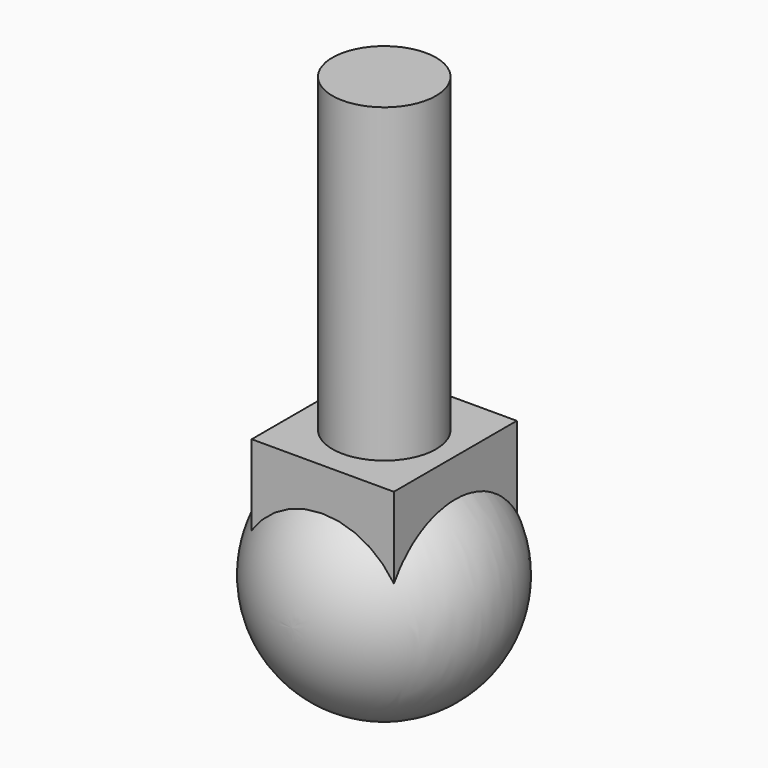
from build123d import *

# Parameters (mm, degrees)
F2_W      = 80.9100866318
F2_H      = 87.9881680012
F5_R      = 35.3495227498
F6_DEPTH  = 299.399793148
F9_W      = 97.0188975334
F9_H      = 104.8525571823
F10_DEPTH = 87.1488675475


# Not quite as in the source:
# - the program builds the solid bodies; features that only make, move or delete a surface that nothing else refers to are left out


with BuildPart() as f1:
    # F0 (on Top) → F1 (revolve)
    with BuildSketch(Plane.XY):
        with BuildLine():
            Line((-0.3210774475, -78.4554468028), (0, 78.4561038017))
            ThreePointArc((0, 78.4561038017), (-78.4559395518, 0.1605390598), (-0.3210774475, -78.4554468028))
        make_face()
    revolve(axis=Axis((-0.1605387237, 0.0003284995, 0), (-0.0020462278, -0.9999979065, 0)))


with BuildPart() as f4:
    # F2 (on Top) → F4 section 0
    with BuildSketch(Plane.XY, mode=Mode.PRIVATE) as f4_s0:
        Rectangle(F2_W, F2_H)
    loft([Vertex(0, 0, 163.5113656521), f4_s0.sketch])


with BuildPart() as f6:
    # F5 (on Top) → F6 (new body)
    with BuildSketch(Plane.XY):
        Circle(F5_R)
    extrude(amount=F6_DEPTH)


with BuildPart() as f8:
    # F7 (on Top) → F8 (revolve)
    with BuildSketch(Plane.XY):
        with BuildLine():
            Line((0, -74.4392126799), (0, 74.4392126799))
            ThreePointArc((0, 74.4392126799), (-74.4392126799, 0), (0, -74.4392126799))
        make_face()
    revolve(axis=Axis((0, 0, 0), (0, -1, 0)))


with BuildPart() as f10:
    # F9 (on Top) → F10 (new body)
    with BuildSketch(Plane.XY):
        Rectangle(F9_W, F9_H)
    extrude(amount=F10_DEPTH)


solid = Compound([f1.part, f4.part, f6.part, f8.part, f10.part])
